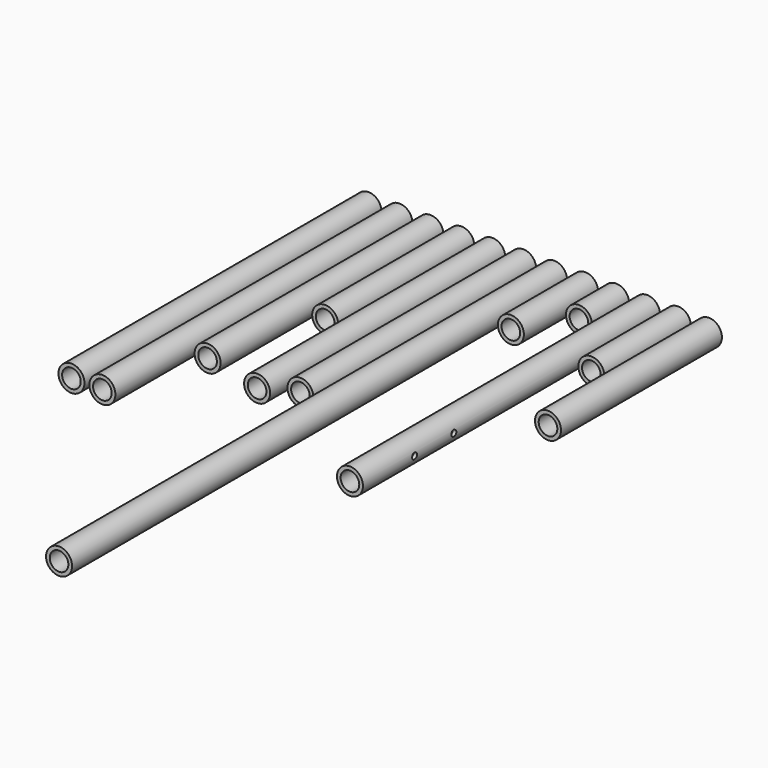
from build123d import *

# Parameters (mm, degrees)
F0_R      = 10.668
F0_R_2    = 7.6454
F1_DEPTH  = 304.8
F2_DEPTH  = 304.8
F3_DEPTH  = 228.6
F4_DEPTH  = 139.7
F5_DEPTH  = 241.3
F6_DEPTH  = 228.6
F7_DEPTH  = 508
F8_DEPTH  = 76.2
F9_DEPTH  = 38.1
F11_DEPTH = 304.8
F12_DEPTH = 88.9
F13_DEPTH = 165.1


with BuildPart() as f1:
    # F0 (on Front) → F1 (new body)
    with BuildSketch(Plane.XZ):
        Circle(F0_R)
        Circle(F0_R_2, mode=Mode.SUBTRACT)
    extrude(amount=F1_DEPTH)


with BuildPart() as f1b:
    # F0 (on Front) → F1, piece 2 (new body)
    with BuildSketch(Plane.XZ):
        with Locations((228.6, 0)):
            Circle(F0_R)
        with Locations((228.6, 0)):
            Circle(F0_R_2, mode=Mode.SUBTRACT)
    extrude(amount=F1_DEPTH)

    # F10 (on Right) → F11 (cut)
    with BuildSketch(Plane.YZ):
        with BuildLine():
            ThreePointArc((-249.2121, 0), (-251.7648, 2.5527), (-254.3175, 0))
            Line((-254.3175, 0), (-249.2121, 0))
        make_face()
        with BuildLine():
            ThreePointArc((-208.9531, 0), (-211.5058, 2.5527), (-214.0585, 0))
            Line((-214.0585, 0), (-208.9531, 0))
        make_face()
        with BuildLine():
            Line((-208.9531, 0), (-214.0585, 0))
            ThreePointArc((-214.0585, 0), (-211.5058, -2.5527), (-208.9531, 0))
        make_face()
        with BuildLine():
            Line((-249.2121, 0), (-254.3175, 0))
            ThreePointArc((-254.3175, 0), (-251.7648, -2.5527), (-249.2121, 0))
        make_face()
    extrude(amount=F11_DEPTH, mode=Mode.SUBTRACT)


with BuildPart() as f2:
    # F0 (on Front) → F2 (new body)
    with BuildSketch(Plane.XZ):
        with Locations((25.4, 0)):
            Circle(F0_R)
        with Locations((25.4, 0)):
            Circle(F0_R_2, mode=Mode.SUBTRACT)
    extrude(amount=F2_DEPTH)


with BuildPart() as f3:
    # F0 (on Front) → F3 (new body)
    with BuildSketch(Plane.XZ):
        with Locations((50.8, 0)):
            Circle(F0_R)
        with Locations((50.8, 0)):
            Circle(F0_R_2, mode=Mode.SUBTRACT)
    extrude(amount=F3_DEPTH)


with BuildPart() as f4:
    # F0 (on Front) → F4 (new body)
    with BuildSketch(Plane.XZ):
        with Locations((76.2, 0)):
            Circle(F0_R)
        with Locations((76.2, 0)):
            Circle(F0_R_2, mode=Mode.SUBTRACT)
    extrude(amount=F4_DEPTH)


with BuildPart() as f5:
    # F0 (on Front) → F5 (new body)
    with BuildSketch(Plane.XZ):
        with Locations((101.6, 0)):
            Circle(F0_R)
        with Locations((101.6, 0)):
            Circle(F0_R_2, mode=Mode.SUBTRACT)
    extrude(amount=F5_DEPTH)


with BuildPart() as f6:
    # F0 (on Front) → F6 (new body)
    with BuildSketch(Plane.XZ):
        with Locations((127, 0)):
            Circle(F0_R)
        with Locations((127, 0)):
            Circle(F0_R_2, mode=Mode.SUBTRACT)
    extrude(amount=F6_DEPTH)


with BuildPart() as f7:
    # F0 (on Front) → F7 (new body)
    with BuildSketch(Plane.XZ):
        with Locations((152.4, 0)):
            Circle(F0_R)
        with Locations((152.4, 0)):
            Circle(F0_R_2, mode=Mode.SUBTRACT)
    extrude(amount=F7_DEPTH)


with BuildPart() as f8:
    # F0 (on Front) → F8 (new body)
    with BuildSketch(Plane.XZ):
        with Locations((177.8, 0)):
            Circle(F0_R)
        with Locations((177.8, 0)):
            Circle(F0_R_2, mode=Mode.SUBTRACT)
    extrude(amount=F8_DEPTH)


with BuildPart() as f9:
    # F0 (on Front) → F9 (new body)
    with BuildSketch(Plane.XZ):
        with Locations((203.2, 0)):
            Circle(F0_R)
        with Locations((203.2, 0)):
            Circle(F0_R_2, mode=Mode.SUBTRACT)
    extrude(amount=F9_DEPTH)


with BuildPart() as f12:
    # F0 (on Front) → F12 (new body)
    with BuildSketch(Plane.XZ):
        with Locations((254, 0)):
            Circle(F0_R)
        with Locations((254, 0)):
            Circle(F0_R_2, mode=Mode.SUBTRACT)
    extrude(amount=F12_DEPTH)


with BuildPart() as f13:
    # F0 (on Front) → F13 (new body)
    with BuildSketch(Plane.XZ):
        with Locations((279.4, 0)):
            Circle(F0_R)
        with Locations((279.4, 0)):
            Circle(F0_R_2, mode=Mode.SUBTRACT)
    extrude(amount=F13_DEPTH)


solid = Compound([f1.part, f1b.part, f2.part, f3.part, f4.part, f5.part, f6.part, f7.part, f8.part, f9.part, f12.part, f13.part])
